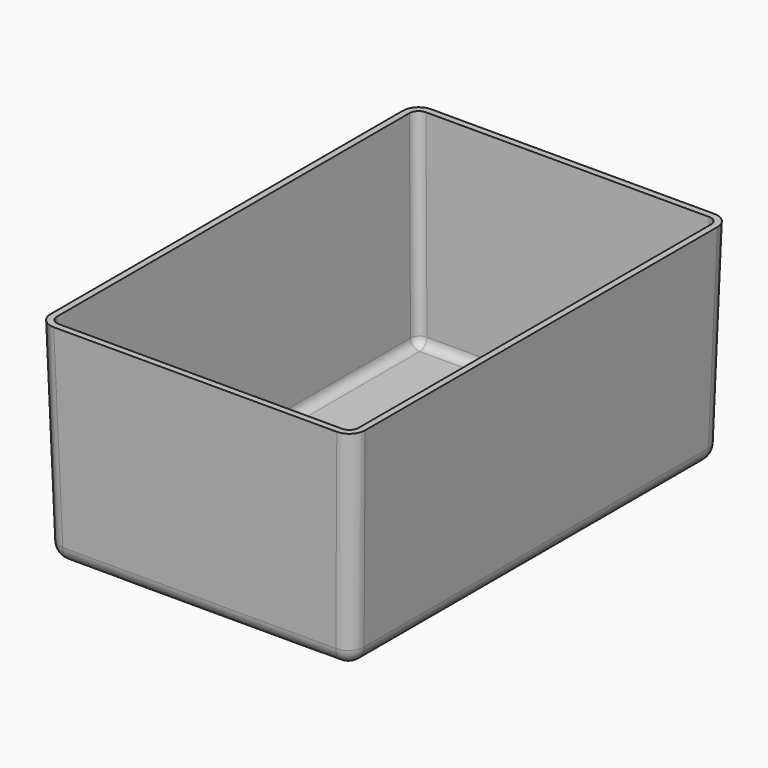
from build123d import *

# Parameters (mm, degrees)
F0_W     = 120
F0_H     = 180
F1_DEPTH = 80
F1_TAPER = 1.5
F2_R     = 6
F3_T     = 2.5
F5_DEPTH = 5
F5_TAPER = -1.5
F6_R     = 1


# Not quite as in the source:
# - a shell that OpenCascade refuses in one call is made with other operations: the cavity is built on its own and cut out


with BuildPart() as f1:
    # F0 (on Top) → F1 (new body)
    with BuildSketch(Plane.XY):
        Rectangle(F0_W, F0_H)
    extrude(amount=-F1_DEPTH, taper=F1_TAPER)

    # F2
    f2_edges = [f1.edges().sort_by_distance(p)[0] for p in [
        (58.952563, -88.952563, -40),
        (-58.952563, -88.952563, -40),
        (58.952563, 88.952563, -40),
        (-58.952563, 88.952563, -40),
        (57.905126, 0, -80),
        (0, 87.905126, -80),
        (-57.905126, 0, -80),
        (0, -87.905126, -80),
    ]]
    fillet(f2_edges, radius=F2_R)

    # F3: shell of thickness 2.5, made by hand


with BuildPart() as f3_core1:
    # F3_t2: copy of F1
    add(f1.part)

    # the walls: a layer under each face that stays
    f3_faces = [f3_core1.faces().sort_by_distance(p)[0] for p in [
        (59.0290644994, 0, -37.0785308449),
        (57.2717058302, -87.2717058302, -37.1110213547),
        (57.2717058302, 87.2717058302, -37.1110213547),
        (56.246927808, 0, -78.2978116605),
        (0, -89.0290644994, -37.0785308449),
        (0, 89.0290644994, -37.0785308449),
        (-57.2717058302, -87.2717058302, -37.1110213547),
        (-57.2717058302, 87.2717058302, -37.1110213547),
        (-59.0290644994, 0, -37.0785308449),
        (55.020659245, -85.0206592509, -78.2978116564),
        (55.020659245, 85.0206592509, -78.2978116564),
        (0, 0, -80),
        (0, -86.246927808, -78.2978116605),
        (0, 86.246927808, -78.2978116605),
        (-55.020659245, -85.0206592509, -78.2978116564),
        (-55.0206592761, 85.0206592452, -78.2978116389),
        (-56.246927808, 0, -78.2978116605),
    ]]
    thicken(f3_faces, amount=-F3_T, mode=Mode.SUBTRACT)


with BuildPart() as f1_1:
    add(f1.part)

    # what is left inside the walls is the cavity
    f3_cavity = [f3_core1.part.solids().sort_by_distance(p)[0] for p in [
        (-26.355263, -17.570173, -0.025),
    ]]
    add(f3_cavity, mode=Mode.SUBTRACT)

    # F4 (on face) → F5 (join)
    with BuildSketch(Plane(origin=(0, 0, -80), x_dir=(1, 0, 0), z_dir=(0, 0, -1))):
        with BuildLine():
            Line((-47.0601850489, 67.0601850489), (-47.0601850489, -67.0601850489))
            ThreePointArc((-47.0601850489, -67.0601850489), (-44.1312528608, -74.1312528608), (-37.0601850489, -77.0601850489))
            Line((-37.0601850489, -77.0601850489), (37.0601850489, -77.0601850489))
            ThreePointArc((37.0601850489, -77.0601850489), (44.1312528608, -74.1312528608), (47.0601850489, -67.0601850489))
            Line((47.0601850489, -67.0601850489), (47.0601850489, 67.0601850489))
            ThreePointArc((47.0601850489, 67.0601850489), (44.1312528608, 74.1312528608), (37.0601850489, 77.0601850489))
            Line((37.0601850489, 77.0601850489), (-37.0601850489, 77.0601850489))
            ThreePointArc((-37.0601850489, 77.0601850489), (-44.1312528608, 74.1312528608), (-47.0601850489, 67.0601850489))
        make_face()
        with BuildLine():
            ThreePointArc((-37.0601850489, -72.0601826906), (-40.5957172873, -70.5957172873), (-42.0601826906, -67.0601850489))
            Line((-42.0601826906, -67.0601850489), (-42.0601826906, 67.0601850489))
            ThreePointArc((-42.0601826906, 67.0601850489), (-40.5957172873, 70.5957172873), (-37.0601850489, 72.0601826906))
            Line((-37.0601850489, 72.0601826906), (37.0601850489, 72.0601826906))
            ThreePointArc((37.0601850489, 72.0601826906), (40.5957172873, 70.5957172873), (42.0601826906, 67.0601850489))
            Line((42.0601826906, 67.0601850489), (42.0601826906, -67.0601850489))
            ThreePointArc((42.0601826906, -67.0601850489), (40.5957172873, -70.5957172873), (37.0601850489, -72.0601826906))
            Line((37.0601850489, -72.0601826906), (-37.0601850489, -72.0601826906))
        make_face(mode=Mode.SUBTRACT)
    extrude(amount=F5_DEPTH, taper=F5_TAPER)

    # F6
    f6_edges = [f1_1.edges().sort_by_distance(p)[0] for p in [
        (-47.060185, 0, -80),
        (-44.223834, 74.223834, -85),
        (0, 71.929253, -85),
        (42.060183, 0, -80),
    ]]
    fillet(f6_edges, radius=F6_R)


solid = f1_1.part
